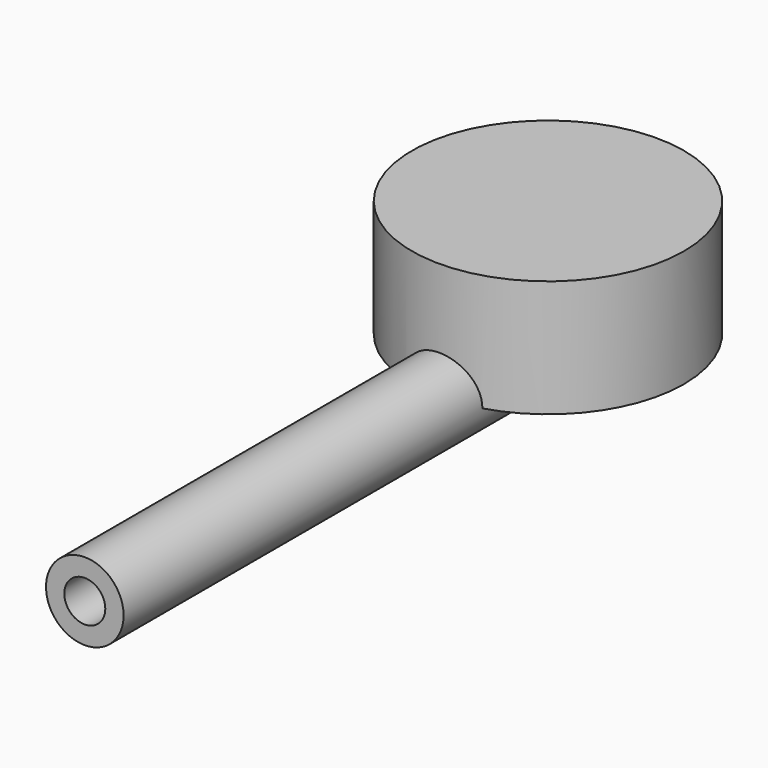
from build123d import *

# Parameters (mm, degrees)
F0_R     = 33.6790507012
F0_R_2   = 17.8010861737
F1_DEPTH = 508
F2_R     = 118.1427595492
F3_DEPTH = 101.6


# Not quite as in the source:
# - the program builds the solid bodies; features that only make, move or delete a surface that nothing else refers to are left out


with BuildPart() as f1:
    # F0 (on Front) → F1 (new body)
    with BuildSketch(Plane.XZ):
        Circle(F0_R)
        Circle(F0_R_2, mode=Mode.SUBTRACT)
    extrude(amount=F1_DEPTH)

    # F2 (on Top) → F3 (join)
    with BuildSketch(Plane.XY):
        with Locations((0, -5.3212568164)):
            Circle(F2_R)
    extrude(amount=F3_DEPTH)


solid = f1.part
